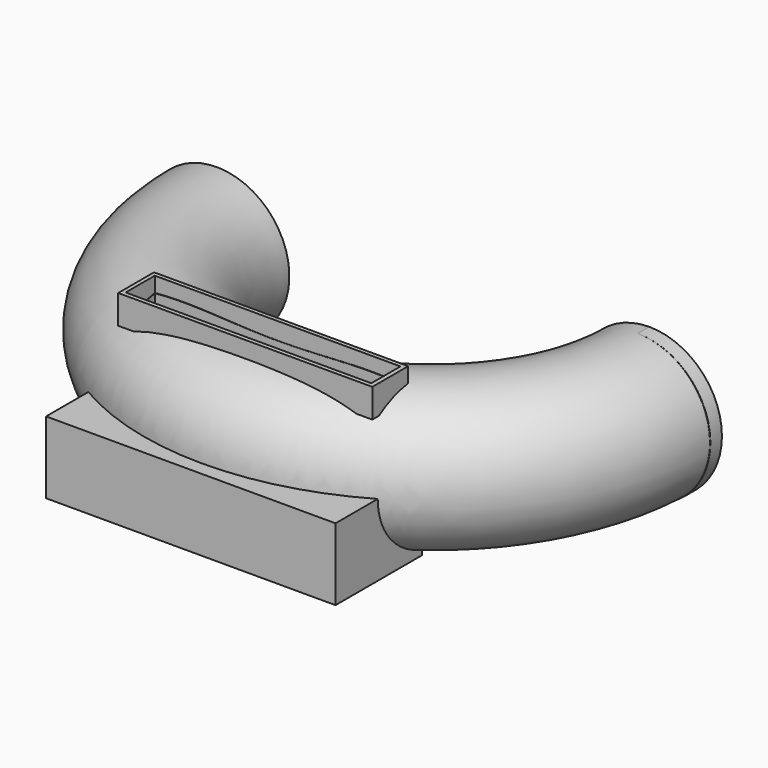
from build123d import *

# Parameters (mm, degrees)
F0_R      = 25.5871618121
F0_R_2    = 20.1441010823
F2_DEPTH  = 5.08
F6_W      = 101.9743236241
F6_H      = 25.4
F7_DEPTH  = 38.1
F8_W      = 89.5350947976
F8_H      = 15.790104866
F8_W_2    = 86.5631140769
F8_H_2    = 12.8241702914
F9_DEPTH  = 10.16
F13_W     = 86.2184539437
F13_H     = 12.5232934952
F14_DEPTH = 17.78


# Not quite as in the source:
# - a feature of the source that left no trace in its solid (it failed there, or was rolled back) is left out


with BuildPart() as f2:
    # F0 (on Front) → F2 (new body)
    with BuildSketch(Plane.XZ):
        Circle(F0_R)
        Circle(F0_R_2, mode=Mode.SUBTRACT)
    extrude(amount=F2_DEPTH)

    # F3: sweep along a path in F1
    with BuildLine(Plane.XY) as f3_path:
        ThreePointArc((-152.4, 0), (-76.2, -76.2), (0, 0))
    # F0 (on Front) → F3 (sweep)
    with BuildSketch(Plane.XZ):
        Circle(F0_R)
        Circle(F0_R_2, mode=Mode.SUBTRACT)
    sweep(path=f3_path.line)

    # F6 (on offset) → F7 (join)
    with BuildSketch(Plane.XZ.offset(106.68)):
        with Locations((-76.2, -12.8871618121)):
            Rectangle(F6_W, F6_H)
    extrude(amount=-F7_DEPTH)

    # F8 (on offset) → F9 (join)
    with BuildSketch(Plane.XY.offset(30.48)):
        with Locations((-76.0538093746, -74.9879702926)):
            Rectangle(F8_W, F8_H)
        with Locations((-76.1367660016, -74.9381892383)):
            Rectangle(F8_W_2, F8_H_2, mode=Mode.SUBTRACT)
    extrude(amount=-F9_DEPTH)

    # F13 (on offset) → F14 (cut)
    with BuildSketch(Plane.XY.offset(30.48)):
        with Locations((-76.1309601367, -74.9482065439)):
            Rectangle(F13_W, F13_H)
    extrude(amount=-F14_DEPTH, mode=Mode.SUBTRACT)


solid = f2.part
